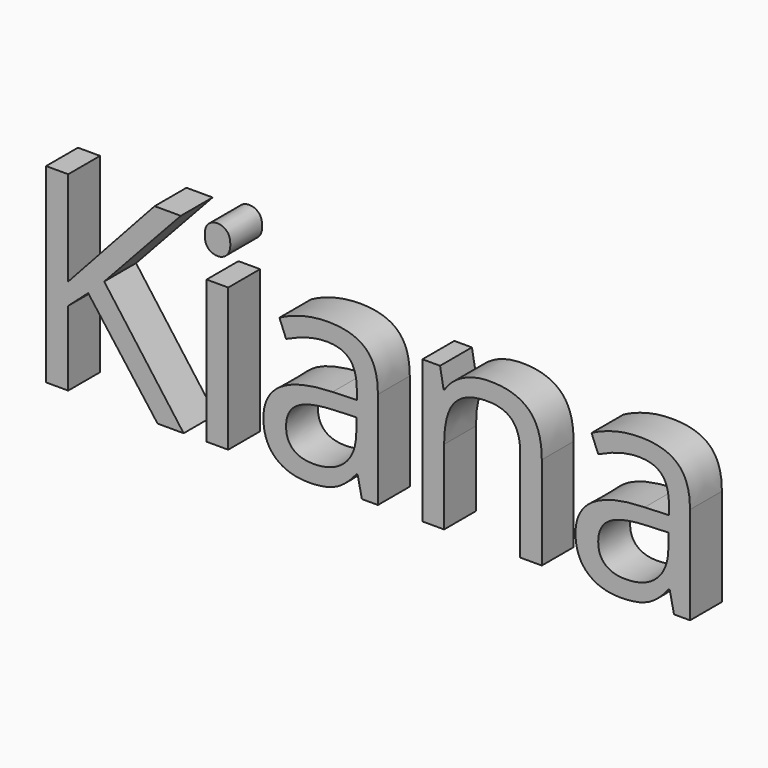
from build123d import *

# Parameters (mm, degrees)
F0_TEXT_SIZE = 170.1855825053
F1_DEPTH     = 25.4


# Not quite as in the source:
# - Text() gives the source's letters only with a copy of the font that has no kerning and outlines rounded to 1/6400 em; it was checked with that copy


with BuildPart() as f1:
    # F0 (on Front) → F1 (new body)
    with BuildSketch(Plane.XZ):
        with Locations((-74.1492062807, -59.1581985354)):
            Text('Kiana', F0_TEXT_SIZE, font='Open Sans', text_align=(TextAlign.LEFT, TextAlign.BOTTOM))
    extrude(amount=F1_DEPTH)


solid = f1.part
